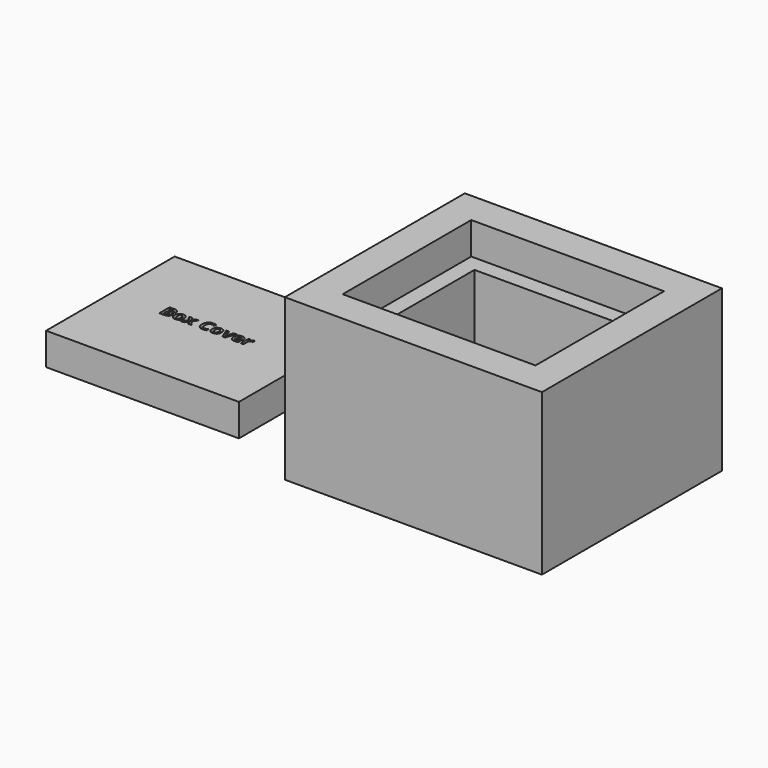
from build123d import *

# Parameters (mm, degrees)
F0_W         = 160
F0_H         = 140
F1_DEPTH     = 100
F2_W         = 120
F2_H         = 100
F3_DEPTH     = 20
F4_W         = 100
F4_H         = 80
F5_DEPTH     = 60
F6_W         = 120
F6_H         = 100
F7_DEPTH     = 20
F8_TEXT_SIZE = 11.1726232186
F9_DEPTH     = 2


# Not quite as in the source:
# - Text() gives the source's letters only with a copy of the font that has no kerning and outlines rounded to 1/6400 em; it was checked with that copy


with BuildPart() as f1:
    # F0 (on Top) → F1 (new body)
    with BuildSketch(Plane.XY):
        Rectangle(F0_W, F0_H)
    extrude(amount=F1_DEPTH)

    # F2 (on face) → F3 (cut)
    with BuildSketch(Plane.XY.offset(100)):
        Rectangle(F2_W, F2_H)
    extrude(amount=-F3_DEPTH, mode=Mode.SUBTRACT)

    # F4 (on face) → F5 (cut)
    with BuildSketch(Plane.XY.offset(80)):
        Rectangle(F4_W, F4_H)
    extrude(amount=-F5_DEPTH, mode=Mode.SUBTRACT)


with BuildPart() as f7:
    # F6 (on Top) → F7 (new body)
    with BuildSketch(Plane.XY):
        with Locations((-184.574007988, 0)):
            Rectangle(F6_W, F6_H)
    extrude(amount=F7_DEPTH)

    # F8 (on face) → F9 (cut)
    with BuildSketch(Plane.XY.offset(20)):
        with Locations((-214.0692150593, -1.2500404755)):
            Text('Box Cover', F8_TEXT_SIZE, font='Open Sans', font_style=FontStyle.BOLD, text_align=(TextAlign.LEFT, TextAlign.BOTTOM))
    extrude(amount=-F9_DEPTH, mode=Mode.SUBTRACT)


solid = Compound([f1.part, f7.part])
